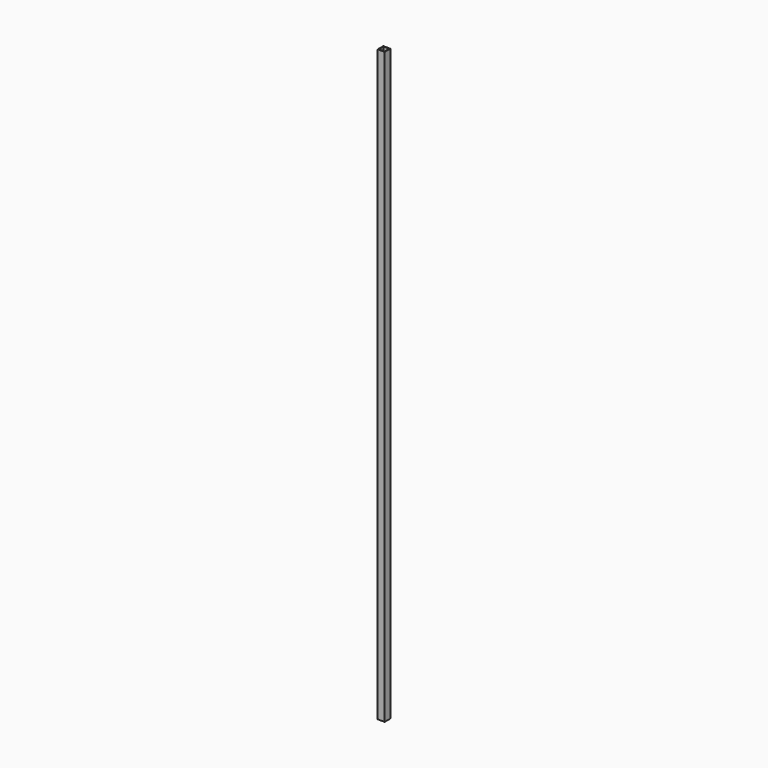
from build123d import *

# Parameters (mm, degrees)
F0_W     = 25.4
F0_H     = 25.4
F0_W_2   = 21.336
F0_H_2   = 21.336
F1_DEPTH = 2133.6


# Not quite as in the source:
# - a feature of the source that left no trace in its solid (it failed there, or was rolled back) is left out


with BuildPart() as f1:
    # F0 (on Top) → F1 (new body)
    with BuildSketch(Plane.XY):
        Rectangle(F0_W, F0_H)
        Rectangle(F0_W_2, F0_H_2, mode=Mode.SUBTRACT)
    extrude(amount=F1_DEPTH)


solid = f1.part
